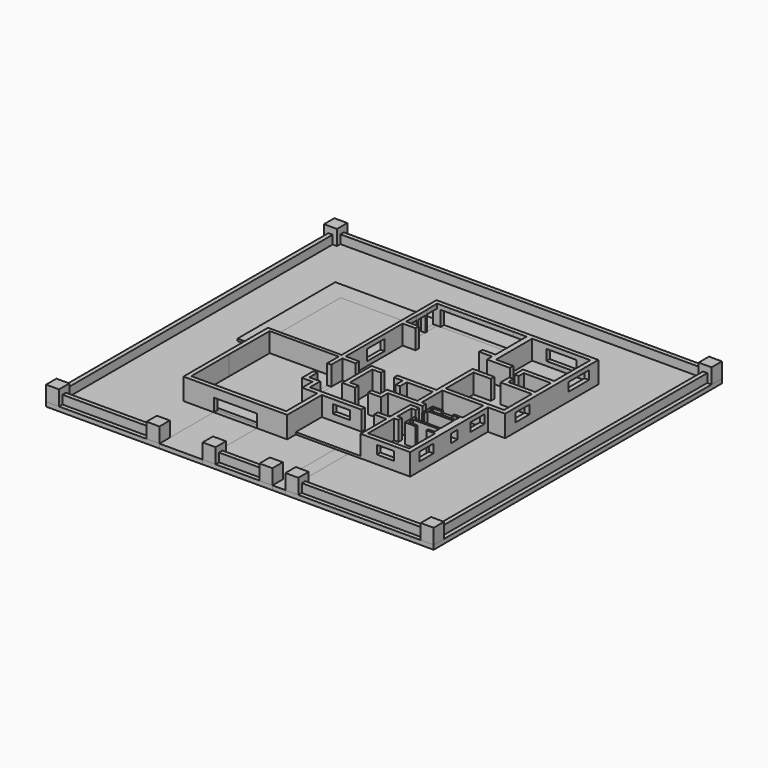
from build123d import *

# Parameters (mm, degrees)
F1_DEPTH  = 254
F2_DEPTH  = 254
F4_DEPTH  = 25.4
F5_W      = 203.2
F5_H      = 177.8
F6_DEPTH  = 50.8
F7_W      = 152.4
F7_H      = 254
F8_DEPTH  = 76.2
F9_W      = 939.5937236786
F9_H      = 25.4
F10_DEPTH = 53.34
F12_DEPTH = 63.5
F14_DEPTH = 76.2
F16_DEPTH = 101.6
F19_DEPTH = 76.2
F21_DEPTH = 76.2
F23_DEPTH = 76.2
F24_W     = 457.2
F24_H     = 177.8
F25_DEPTH = 76.2
F27_DEPTH = 76.2
F28_W     = 25.4
F28_H     = 50.8
F29_DEPTH = 50.8
F30_W     = 4055.1800727844
F30_H     = 3734.5069646835
F31_DEPTH = 50.8
F33_W     = 762
F33_H     = 1016
F34_DEPTH = 76.2
F35_W     = 762
F35_H     = 1016
F36_DEPTH = 76.2
F37_W     = 762
F37_H     = 1016
F38_DEPTH = 50.8
F39_DEPTH = 25.4
F40_DEPTH = 508
F41_DEPTH = 254
F42_DEPTH = 254
F45_DEPTH = 381
F46_W     = 152.4
F46_H     = 50.8
F47_DEPTH = 1016
F48_DEPTH = 1016
F49_W     = 152.4
F49_H     = 152.4
F50_DEPTH = 177.8
F52_DEPTH = 1524
F53_W     = 152.4
F53_H     = 152.4
F54_DEPTH = 177.8
F55_W     = 152.4
F55_H     = 152.4
F56_DEPTH = 177.8
F58_DEPTH = 3937
F60_DEPTH = 4318
F62_DEPTH = 4064
F65_DEPTH = 1905
F66_DEPTH = 1905
F67_DEPTH = 799.465
F68_W     = 508
F68_H     = 152.4
F69_DEPTH = 76.2
F70_W     = 152.4
F70_H     = 152.4
F71_DEPTH = 177.8
F72_DEPTH = 1143
F74_DEPTH = 635


with BuildPart() as f1:
    # F0 (on Top) → F1 (new body)
    with BuildSketch(Plane.XY):
        Polygon((177.8, 1192.7142027378), (-304.8, 1192.7142027378), (-635, 1192.7142027378), (-635, 508), (-635, -51.8857972622), (-47.8687277794, -51.8857972622), (587.1312722206, -51.8857972622), (587.1312722206, 456.1142027378), (1349.1312722206, 456.1142027378), (1349.1312722206, 75.1142027378), (1933.3312722206, 75.1142027378), (1933.3312722206, 1218.1142027378), (2136.5312722206, 1218.1142027378), (2136.5312722206, 2589.7142027378), (1349.1312722206, 2589.7142027378), (1179.474234581, 2589.7142027378), (431.8, 2589.7142027378), (231.5312722206, 2589.7142027378), (231.5312722206, 2081.7142027378), (231.5312722206, 1192.7142027378), align=None)
        Polygon((533.4, 0), (0, 0), (-584.2, 0), (-584.2, 558.8), (-581.2687277794, 1150.6002895355), (-301.8687277794, 1150.6002895355), (231.5312722206, 1150.6002895355), (231.5312722206, 608.5142027378), (355.6, 608.5142027378), (355.6, 456.1142027378), (482.6, 456.1142027378), (533.4, 456.1142027378), align=None, mode=Mode.SUBTRACT)
        Polygon((1396.7937236786, 127), (1396.7937236786, 508), (1447.5937236786, 508), (1447.5937236786, 558.8), (1396.7937236786, 558.8), (1396.7937236786, 762), (1447.5937236786, 762), (1447.5937236786, 812.8), (1396.7937236786, 812.8), (1345.9937236786, 812.8), (1345.9937236786, 762), (1345.9937236786, 508), (1041.1937236786, 508), (533.4, 508), (406.4, 508), (406.4, 660.4), (279.4, 660.4), (279.4, 1143), (437.7339612484, 1143), (437.7339612484, 1193.8), (279.4, 1193.8), (279.4, 2032), (431.8, 2032), (431.8, 2081.7142027378), (279.4, 2081.7142027378), (279.4, 2538.9142027378), (431.8, 2538.9142027378), (1179.474234581, 2540), (1331.874234581, 2540), (1331.874234581, 2081.7142027378), (1179.474234581, 2081.7142027378), (1179.474234581, 2032), (1331.874234581, 2032), (1331.874234581, 1957.4247688293), (1600.2, 1957.4247688293), (1600.2, 2008.2247688293), (1396.7937236786, 2008.2247688293), (1396.7937236786, 2540), (2082.5937236786, 2540), (2082.5937236786, 2008.2247688293), (1714.5, 2008.2247688293), (1714.5, 1957.4247688293), (1714.5, 1881.2247688293), (1765.3, 1881.2247688293), (1765.3, 1957.4247688293), (2082.5937236786, 1957.4247688293), (2082.5937236786, 1728.8247688293), (1765.3, 1728.8247688293), (1765.3, 1805.0247688293), (1714.5, 1805.0247688293), (1714.5, 1728.8247688293), (1714.5, 1678.0247688293), (2082.5937236786, 1678.0247688293), (2082.5937236786, 1270), (1828.5937236786, 1270), (1396.7937236786, 1270), (1396.7937236786, 1678.0247688293), (1600.2, 1678.0247688293), (1600.2, 1728.8247688293), (1345.9937236786, 1728.8247688293), (1345.9937236786, 1574.8), (1345.9937236786, 1320.8), (1345.9937236786, 1270), (1345.9937236786, 1193.8), (1193.5937236786, 1193.8), (1039.9870965004, 1193.8), (887.5870965004, 1193.8), (887.5870965004, 1143), (989.1870965004, 1143), (989.1870965004, 1041.4), (1039.9870965004, 1041.4), (1039.9870965004, 1143), (1193.5937236786, 1143), (1345.9937236786, 1143), (1345.9937236786, 1117.6073976807), (1345.9937236786, 939.8), (1345.9937236786, 914.4), (1039.9870965004, 914.4), (989.1870965004, 914.4), (989.1870965004, 812.8), (938.3870965004, 812.8), (887.5870965004, 812.8), (887.5870965004, 762), (1039.9870965004, 762), (1039.9870965004, 812.8), (1039.9870965004, 863.6), (1345.9937236786, 863.6), (1396.7937236786, 863.6), (1447.5937236786, 863.6), (1447.5937236786, 914.4), (1396.7937236786, 914.4), (1396.7937236786, 965.2), (1396.7937236786, 1219.2), (1828.5937236786, 1219.2), (1879.3937236786, 1219.2), (1879.3937236786, 914.4), (1879.3937236786, 811.3352970581), (1879.3937236786, 749.310195446), (1879.3937236786, 508), (1879.3937236786, 127), align=None, mode=Mode.SUBTRACT)
        Polygon((1777.7937236786, 508), (1879.3937236786, 508), (1879.3937236786, 749.310195446), (1879.3937236786, 811.3352970581), (1879.3937236786, 914.4), (1777.7937236786, 914.4), (1777.7937236786, 889), (1853.9937236786, 889), (1853.9937236786, 838.2), (1549.1937236786, 838.2), (1549.1937236786, 889), (1650.7937236786, 889), (1650.7937236786, 914.4), (1523.7937236786, 914.4), (1523.7937236786, 863.6), (1523.7937236786, 811.3352970581), (1523.7937236786, 757.4872970581), (1549.1937236786, 757.4872970581), (1549.1937236786, 811.3352970581), (1853.9937236786, 811.3352970581), (1853.9937236786, 622.3084970581), (1549.1937236786, 622.3084970581), (1549.1937236786, 650.748), (1523.7937236786, 650.748), (1523.7937236786, 596.9), (1523.7937236786, 508), (1650.7937236786, 508), (1650.7937236786, 533.4), (1549.1937236786, 533.4), (1549.1937236786, 596.9), (1853.9937236786, 596.9), (1853.9937236786, 533.4), (1777.7937236786, 533.4), align=None)
    extrude(amount=F1_DEPTH)

    # F0 (on Top) → F2 (join)
    with BuildSketch(Plane.XY):
        Polygon((177.8, 1192.7142027378), (-304.8, 1192.7142027378), (-635, 1192.7142027378), (-635, 508), (-635, -51.8857972622), (-47.8687277794, -51.8857972622), (587.1312722206, -51.8857972622), (587.1312722206, 456.1142027378), (1349.1312722206, 456.1142027378), (1349.1312722206, 75.1142027378), (1933.3312722206, 75.1142027378), (1933.3312722206, 1218.1142027378), (2136.5312722206, 1218.1142027378), (2136.5312722206, 2589.7142027378), (1349.1312722206, 2589.7142027378), (1179.474234581, 2589.7142027378), (431.8, 2589.7142027378), (231.5312722206, 2589.7142027378), (231.5312722206, 2081.7142027378), (231.5312722206, 1192.7142027378), align=None)
        Polygon((533.4, 0), (0, 0), (-584.2, 0), (-584.2, 558.8), (-581.2687277794, 1150.6002895355), (-301.8687277794, 1150.6002895355), (231.5312722206, 1150.6002895355), (231.5312722206, 608.5142027378), (355.6, 608.5142027378), (355.6, 456.1142027378), (482.6, 456.1142027378), (533.4, 456.1142027378), align=None, mode=Mode.SUBTRACT)
        Polygon((1396.7937236786, 127), (1396.7937236786, 508), (1447.5937236786, 508), (1447.5937236786, 558.8), (1396.7937236786, 558.8), (1396.7937236786, 762), (1447.5937236786, 762), (1447.5937236786, 812.8), (1396.7937236786, 812.8), (1345.9937236786, 812.8), (1345.9937236786, 762), (1345.9937236786, 508), (1041.1937236786, 508), (533.4, 508), (406.4, 508), (406.4, 660.4), (279.4, 660.4), (279.4, 1143), (437.7339612484, 1143), (437.7339612484, 1193.8), (279.4, 1193.8), (279.4, 2032), (431.8, 2032), (431.8, 2081.7142027378), (279.4, 2081.7142027378), (279.4, 2538.9142027378), (431.8, 2538.9142027378), (1179.474234581, 2540), (1331.874234581, 2540), (1331.874234581, 2081.7142027378), (1179.474234581, 2081.7142027378), (1179.474234581, 2032), (1331.874234581, 2032), (1331.874234581, 1957.4247688293), (1600.2, 1957.4247688293), (1600.2, 2008.2247688293), (1396.7937236786, 2008.2247688293), (1396.7937236786, 2540), (2082.5937236786, 2540), (2082.5937236786, 2008.2247688293), (1714.5, 2008.2247688293), (1714.5, 1957.4247688293), (1714.5, 1881.2247688293), (1765.3, 1881.2247688293), (1765.3, 1957.4247688293), (2082.5937236786, 1957.4247688293), (2082.5937236786, 1728.8247688293), (1765.3, 1728.8247688293), (1765.3, 1805.0247688293), (1714.5, 1805.0247688293), (1714.5, 1728.8247688293), (1714.5, 1678.0247688293), (2082.5937236786, 1678.0247688293), (2082.5937236786, 1270), (1828.5937236786, 1270), (1396.7937236786, 1270), (1396.7937236786, 1678.0247688293), (1600.2, 1678.0247688293), (1600.2, 1728.8247688293), (1345.9937236786, 1728.8247688293), (1345.9937236786, 1574.8), (1345.9937236786, 1320.8), (1345.9937236786, 1270), (1345.9937236786, 1193.8), (1193.5937236786, 1193.8), (1039.9870965004, 1193.8), (887.5870965004, 1193.8), (887.5870965004, 1143), (989.1870965004, 1143), (989.1870965004, 1041.4), (1039.9870965004, 1041.4), (1039.9870965004, 1143), (1193.5937236786, 1143), (1345.9937236786, 1143), (1345.9937236786, 1117.6073976807), (1345.9937236786, 939.8), (1345.9937236786, 914.4), (1039.9870965004, 914.4), (989.1870965004, 914.4), (989.1870965004, 812.8), (938.3870965004, 812.8), (887.5870965004, 812.8), (887.5870965004, 762), (1039.9870965004, 762), (1039.9870965004, 812.8), (1039.9870965004, 863.6), (1345.9937236786, 863.6), (1396.7937236786, 863.6), (1447.5937236786, 863.6), (1447.5937236786, 914.4), (1396.7937236786, 914.4), (1396.7937236786, 965.2), (1396.7937236786, 1219.2), (1828.5937236786, 1219.2), (1879.3937236786, 1219.2), (1879.3937236786, 914.4), (1879.3937236786, 811.3352970581), (1879.3937236786, 749.310195446), (1879.3937236786, 508), (1879.3937236786, 127), align=None, mode=Mode.SUBTRACT)
    extrude(amount=F2_DEPTH)

    # F5 (on face) → F6 (cut)
    with BuildSketch(Plane(origin=(231.5312722206, 0, 0), x_dir=(0, -1, 0), z_dir=(-1, 0, 0))):
        Polygon((-777.9572461367, 203.2), (-777.9572461367, 254), (-879.5572461367, 254), (-981.1572461367, 254), (-981.1572461367, 203.2), align=None)
        with Locations((-879.5572461367, 114.3)):
            Rectangle(F5_W, F5_H)
    extrude(amount=-F6_DEPTH, mode=Mode.SUBTRACT)

    # F7 (on face) → F8 (cut)
    with BuildSketch(Plane.XZ.offset(-456.1142027378)):
        with Locations((1128.791085434, 127)):
            Rectangle(F7_W, F7_H)
    extrude(amount=-F8_DEPTH, mode=Mode.SUBTRACT)

    # F11 (on face) → F12 (cut)
    with BuildSketch(Plane.XZ.offset(-456.1142027378)):
        Polygon((921.4611788273, 203.2), (819.8611788273, 203.2), (718.2611788273, 203.2), (718.2611788273, 101.6), (921.4611788273, 101.6), align=None)
    extrude(amount=-F12_DEPTH, mode=Mode.SUBTRACT)

    # F13 (on face) → F14 (cut)
    with BuildSketch(Plane.XZ.offset(-75.1142027378)):
        Polygon((1742.8312722206, 203.2), (1641.2312722206, 203.2), (1539.6312722206, 203.2), (1539.6312722206, 101.6), (1742.8312722206, 101.6), align=None)
    extrude(amount=-F14_DEPTH, mode=Mode.SUBTRACT)

    # F15 (on face) → F16 (cut)
    with BuildSketch(Plane.YZ.offset(1933.3312722206)):
        Polygon((418.0142027378, 203.2), (316.4142027378, 203.2), (214.8142027378, 203.2), (214.8142027378, 101.6), (418.0142027378, 101.6), align=None)
        Polygon((1167.3142027378, 203.2), (1065.7142027378, 203.2), (964.1142027378, 203.2), (964.1142027378, 101.6), (1167.3142027378, 101.6), align=None)
        Polygon((773.6142027378, 203.2), (710.1142027378, 203.2), (672.0142027378, 203.2), (672.0142027378, 101.6), (773.6142027378, 101.6), align=None)
    extrude(amount=-F16_DEPTH, mode=Mode.SUBTRACT)

    # F18 (on face) → F19 (cut)
    with BuildSketch(Plane.YZ.offset(2136.5312722206)):
        Polygon((2452.1544022799, 203.2), (2299.7544022799, 203.2), (2147.3544022799, 203.2), (2147.3544022799, 101.6), (2452.1544022799, 101.6), align=None)
        Polygon((1573.7142027378, 203.2), (1472.1142027378, 203.2), (1370.5142027378, 203.2), (1370.5142027378, 101.6), (1573.7142027378, 101.6), align=None)
    extrude(amount=-F19_DEPTH, mode=Mode.SUBTRACT)

    # F20 (on face) → F21 (cut)
    with BuildSketch(Plane(origin=(0, 2589.7142027378, 0), x_dir=(-1, 0, 0), z_dir=(0, 1, 0))):
        Polygon((-1565.0312722206, 203.2), (-1742.8312722206, 203.2), (-1920.6312722206, 203.2), (-1920.6312722206, 76.2), (-1565.0312722206, 76.2), align=None)
    extrude(amount=-F21_DEPTH, mode=Mode.SUBTRACT)

    # F22 (on face) → F23 (cut)
    with BuildSketch(Plane(origin=(0, 2589.7142027378, 0), x_dir=(-1, 0, 0), z_dir=(0, 1, 0))):
        Polygon((-320.4312722206, 203.2), (-803.0312722206, 203.2), (-1285.6312722206, 203.2), (-1285.6312722206, 25.4), (-320.4312722206, 25.4), align=None)
    extrude(amount=-F23_DEPTH, mode=Mode.SUBTRACT)

    # F24 (on face) → F25 (cut)
    with BuildSketch(Plane(origin=(231.5312722206, 0, 0), x_dir=(0, -1, 0), z_dir=(-1, 0, 0))):
        with Locations((-2310.3142027378, 114.3)):
            Rectangle(F24_W, F24_H)
    extrude(amount=-F25_DEPTH, mode=Mode.SUBTRACT)

    # F26 (on face) → F27 (cut)
    with BuildSketch(Plane(origin=(231.5312722206, 0, 0), x_dir=(0, -1, 0), z_dir=(-1, 0, 0))):
        Polygon((-1510.2142027378, 203.2), (-1764.2142027378, 203.2), (-1764.2142027378, 76.2), (-1637.2142027378, 76.2), (-1510.2142027378, 76.2), align=None)
    extrude(amount=-F27_DEPTH, mode=Mode.SUBTRACT)



with BuildPart() as f2:
    # F0 (on Top) → F2, piece 2 (new body)
    with BuildSketch(Plane.XY):
        Polygon((582.7870965004, 762), (735.1870965004, 762), (735.1870965004, 812.8), (633.5870965004, 812.8), (633.5870965004, 1143), (735.1870965004, 1143), (735.1870965004, 1193.8), (582.7870965004, 1193.8), (582.7870965004, 1143), (582.7870965004, 812.8), align=None)
    extrude(amount=F2_DEPTH)


with BuildPart() as f4:
    # F3 (on face) → F4 (new body)
    with BuildSketch(Plane(origin=(0, 0, 0), x_dir=(1, 0, 0), z_dir=(0, 0, -1))):
        Polygon((533.4, -456.1142027378), (533.4, 0), (-584.2, 0), (-584.2, -558.8), (-581.2687277794, -1150.6002895355), (231.5312722206, -1150.6002895355), (231.5312722206, -608.5142027378), (355.6, -608.5142027378), (355.6, -456.1142027378), align=None)
    extrude(amount=-F4_DEPTH)


with BuildPart() as f4b:
    # F3 (on face) → F4, piece 2 (new body)
    with BuildSketch(Plane(origin=(0, 0, 0), x_dir=(1, 0, 0), z_dir=(0, 0, -1))):
        Polygon((1039.9870965004, -762), (1039.9870965004, -863.6), (1447.5937236786, -863.6), (1447.5937236786, -914.4), (1396.7937236786, -914.4), (1396.7937236786, -1219.2), (1879.3937236786, -1219.2), (1879.3937236786, -914.4), (1777.7937236786, -914.4), (1777.7937236786, -889), (1853.9937236786, -889), (1853.9937236786, -838.2), (1549.1937236786, -838.2), (1549.1937236786, -889), (1650.7937236786, -889), (1650.7937236786, -914.4), (1523.7937236786, -914.4), (1523.7937236786, -757.4872970581), (1549.1937236786, -757.4872970581), (1549.1937236786, -811.3352970581), (1853.9937236786, -811.3352970581), (1853.9937236786, -622.3084970581), (1549.1937236786, -622.3084970581), (1549.1937236786, -650.748), (1523.7937236786, -650.748), (1523.7937236786, -508), (1650.7937236786, -508), (1650.7937236786, -533.4), (1549.1937236786, -533.4), (1549.1937236786, -596.9), (1853.9937236786, -596.9), (1853.9937236786, -533.4), (1777.7937236786, -533.4), (1777.7937236786, -508), (1879.3937236786, -508), (1879.3937236786, -127), (1396.7937236786, -127), (1396.7937236786, -508), (1447.5937236786, -508), (1447.5937236786, -558.8), (1396.7937236786, -558.8), (1396.7937236786, -762), (1447.5937236786, -762), (1447.5937236786, -812.8), (1345.9937236786, -812.8), (1345.9937236786, -508), (406.4, -508), (406.4, -660.4), (279.4, -660.4), (279.4, -1143), (437.7339612484, -1143), (437.7339612484, -1193.8), (279.4, -1193.8), (279.4, -2032), (431.8, -2032), (431.8, -2081.7142027378), (279.4, -2081.7142027378), (279.4, -2538.9142027378), (431.8, -2538.9142027378), (1179.474234581, -2540), (1331.874234581, -2540), (1331.874234581, -2081.7142027378), (1179.474234581, -2081.7142027378), (1179.474234581, -2032), (1331.874234581, -2032), (1331.874234581, -1957.4247688293), (1600.2, -1957.4247688293), (1600.2, -2008.2247688293), (1396.7937236786, -2008.2247688293), (1396.7937236786, -2540), (2082.5937236786, -2540), (2082.5937236786, -2008.2247688293), (1714.5, -2008.2247688293), (1714.5, -1881.2247688293), (1765.3, -1881.2247688293), (1765.3, -1957.4247688293), (2082.5937236786, -1957.4247688293), (2082.5937236786, -1728.8247688293), (1765.3, -1728.8247688293), (1765.3, -1805.0247688293), (1714.5, -1805.0247688293), (1714.5, -1678.0247688293), (2082.5937236786, -1678.0247688293), (2082.5937236786, -1270), (1396.7937236786, -1270), (1396.7937236786, -1678.0247688293), (1600.2, -1678.0247688293), (1600.2, -1728.8247688293), (1345.9937236786, -1728.8247688293), (1345.9937236786, -1193.8), (887.5870965004, -1193.8), (887.5870965004, -1143), (989.1870965004, -1143), (989.1870965004, -1041.4), (1039.9870965004, -1041.4), (1039.9870965004, -1143), (1345.9937236786, -1143), (1345.9937236786, -914.4), (989.1870965004, -914.4), (989.1870965004, -812.8), (887.5870965004, -812.8), (887.5870965004, -762), align=None)
    extrude(amount=-F4_DEPTH)


with BuildPart() as f10:
    # F9 (on face) → F10 (new body)
    with BuildSketch(Plane.XZ.offset(-508)):
        with Locations((876.1968618393, 12.7)):
            Rectangle(F9_W, F9_H)
    extrude(amount=F10_DEPTH)


with BuildPart() as f29:
    # F28 (on face) → F29 (new body)
    with BuildSketch(Plane(origin=(231.5312722206, 0, 0), x_dir=(0, -1, 0), z_dir=(-1, 0, 0))):
        Polygon((-2361.1142027378, 254), (-2361.1142027378, 203.2), (-2310.3142027378, 203.2), (-2259.5142027378, 203.2), (-2259.5142027378, 254), align=None)
        Polygon((-2361.1142027378, 25.4), (-2361.1142027378, 203.2), (-2386.5142027378, 203.2), (-2386.5142027378, 0), (-2259.5142027378, 0), (-2259.5142027378, 25.4), (-2310.3142027378, 25.4), align=None)
        with Locations((-2373.8142027378, 228.6)):
            Rectangle(F28_W, F28_H)
        with Locations((-2246.8142027378, 228.6)):
            Rectangle(F28_W, F28_H)
        Polygon((-2234.1142027378, 203.2), (-2259.5142027378, 203.2), (-2259.5142027378, 25.4), (-2259.5142027378, 0), (-2234.1142027378, 0), align=None)
    extrude(amount=-F29_DEPTH)


with BuildPart() as f31:
    # F30 (on face) → F31 (new body)
    with BuildSketch(Plane(origin=(0, 0, 0), x_dir=(1, 0, 0), z_dir=(0, 0, -1))):
        with Locations((922.8382110596, -1270.1082825661)):
            Rectangle(F30_W, F30_H)
        Polygon((2136.5312722206, -2589.7142027378), (231.5312722206, -2589.7142027378), (231.5312722206, -1192.7142027378), (-635, -1192.7142027378), (-635, 51.8857972622), (587.1312722206, 51.8857972622), (587.1312722206, -456.1142027378), (1052.591085434, -456.1142027378), (1052.591085434, -508), (406.4, -508), (406.4, -660.4), (279.4, -660.4), (279.4, -1143), (437.7339612484, -1143), (437.7339612484, -1193.8), (279.4, -1193.8), (279.4, -2032), (431.8, -2032), (431.8, -2081.7142027378), (279.4, -2081.7142027378), (279.4, -2538.9142027378), (431.8, -2538.9142027378), (1179.474234581, -2540), (1331.874234581, -2540), (1331.874234581, -2081.7142027378), (1179.474234581, -2081.7142027378), (1179.474234581, -2032), (1331.874234581, -2032), (1331.874234581, -1957.4247688293), (1600.2, -1957.4247688293), (1600.2, -2008.2247688293), (1396.7937236786, -2008.2247688293), (1396.7937236786, -2540), (2082.5937236786, -2540), (2082.5937236786, -2008.2247688293), (1714.5, -2008.2247688293), (1714.5, -1881.2247688293), (1765.3, -1881.2247688293), (1765.3, -1957.4247688293), (2082.5937236786, -1957.4247688293), (2082.5937236786, -1728.8247688293), (1765.3, -1728.8247688293), (1765.3, -1805.0247688293), (1714.5, -1805.0247688293), (1714.5, -1678.0247688293), (2082.5937236786, -1678.0247688293), (2082.5937236786, -1270), (1396.7937236786, -1270), (1396.7937236786, -1678.0247688293), (1600.2, -1678.0247688293), (1600.2, -1728.8247688293), (1345.9937236786, -1728.8247688293), (1345.9937236786, -1193.8), (887.5870965004, -1193.8), (887.5870965004, -1143), (989.1870965004, -1143), (989.1870965004, -1041.4), (1039.9870965004, -1041.4), (1039.9870965004, -1143), (1345.9937236786, -1143), (1345.9937236786, -914.4), (989.1870965004, -914.4), (989.1870965004, -812.8), (887.5870965004, -812.8), (887.5870965004, -762), (1039.9870965004, -762), (1039.9870965004, -863.6), (1447.5937236786, -863.6), (1447.5937236786, -914.4), (1396.7937236786, -914.4), (1396.7937236786, -1219.2), (1879.3937236786, -1219.2), (1879.3937236786, -914.4), (1777.7937236786, -914.4), (1777.7937236786, -889), (1853.9937236786, -889), (1853.9937236786, -838.2), (1549.1937236786, -838.2), (1549.1937236786, -889), (1650.7937236786, -889), (1650.7937236786, -914.4), (1523.7937236786, -914.4), (1523.7937236786, -757.4872970581), (1549.1937236786, -757.4872970581), (1549.1937236786, -811.3352970581), (1853.9937236786, -811.3352970581), (1853.9937236786, -622.3084970581), (1549.1937236786, -622.3084970581), (1549.1937236786, -650.748), (1523.7937236786, -650.748), (1523.7937236786, -508), (1650.7937236786, -508), (1650.7937236786, -533.4), (1549.1937236786, -533.4), (1549.1937236786, -596.9), (1853.9937236786, -596.9), (1853.9937236786, -533.4), (1777.7937236786, -533.4), (1777.7937236786, -508), (1879.3937236786, -508), (1879.3937236786, -127), (1396.7937236786, -127), (1396.7937236786, -508), (1447.5937236786, -508), (1447.5937236786, -558.8), (1396.7937236786, -558.8), (1396.7937236786, -762), (1447.5937236786, -762), (1447.5937236786, -812.8), (1345.9937236786, -812.8), (1345.9937236786, -508), (1204.991085434, -508), (1204.991085434, -456.1142027378), (1349.1312722206, -456.1142027378), (1349.1312722206, -75.1142027378), (1933.3312722206, -75.1142027378), (1933.3312722206, -1218.1142027378), (2136.5312722206, -1218.1142027378), align=None, mode=Mode.SUBTRACT)
    extrude(amount=F31_DEPTH)

    # F33 (on face) → F34 (cut)
    with BuildSketch(Plane.XY):
        with Locations((-381, 1911.4676551819)):
            Rectangle(F33_W, F33_H)
    extrude(amount=-F34_DEPTH, mode=Mode.SUBTRACT)

    # F40 (add): a face of the model
    f40_faces = [f31.faces().sort_by_distance(p)[0] for p in [
        (-1104.7518253326, 1270.1082825661, -25.4),
    ]]
    extrude(f40_faces, amount=F40_DEPTH)

    # F41 (add): a face of the model
    f41_faces = [f31.faces().sort_by_distance(p)[0] for p in [
        (668.8382110596, -597.1451997757, -25.4),
    ]]
    extrude(f41_faces, amount=F41_DEPTH)

    # F42 (add): a face of the model
    f42_faces = [f31.faces().sort_by_distance(p)[0] for p in [
        (668.8382110596, 3137.3617649078, -25.4),
    ]]
    extrude(f42_faces, amount=F42_DEPTH)

    # F46 (on face) → F47 (cut)
    with BuildSketch(Plane.XZ.offset(851.1451997757)):
        with Locations((1128.791085434, -25.4)):
            Rectangle(F46_W, F46_H)
    extrude(amount=-F47_DEPTH, mode=Mode.SUBTRACT)


with BuildPart() as f31b:
    # F30 (on face) → F31, piece 2 (new body)
    with BuildSketch(Plane(origin=(0, 0, 0), x_dir=(1, 0, 0), z_dir=(0, 0, -1))):
        Polygon((533.4, -456.1142027378), (533.4, 0), (-584.2, 0), (-584.2, -558.8), (-581.2687277794, -1150.6002895355), (231.5312722206, -1150.6002895355), (231.5312722206, -608.5142027378), (355.6, -608.5142027378), (355.6, -456.1142027378), align=None)
    extrude(amount=F31_DEPTH)


with BuildPart() as f36:
    # F35 (on face) → F36 (new body)
    with BuildSketch(Plane(origin=(0, 0, -50.8), x_dir=(1, 0, 0), z_dir=(0, 0, -1))):
        with Locations((-381, -1911.4676551819)):
            Rectangle(F35_W, F35_H)
    extrude(amount=-F36_DEPTH)


with BuildPart() as f38:
    # F37 (on face) → F38 (new body)
    with BuildSketch(Plane.XY):
        Polygon((231.5312722206, 1192.7142027378), (231.5312722206, 2589.7142027378), (231.5312722206, 2630.2114551819), (-993.521, 2630.2114551819), (-993.521, 2419.4676551819), (-993.521, 1192.7142027378), (-762, 1192.7142027378), (-635, 1192.7142027378), align=None)
        with Locations((-381, 1911.4676551819)):
            Rectangle(F37_W, F37_H, mode=Mode.SUBTRACT)
    extrude(amount=-F38_DEPTH)


with BuildPart() as f39:
    # F39 (new): a face of the model
    f39_faces = [f38.part.faces().sort_by_distance(p)[0] for p in [
        (212.6443682381, 1911.4628289598, 0),
    ]]
    extrude(f39_faces, amount=F39_DEPTH)


with BuildPart() as f45:
    # F44 (on face) → F45 (new body)
    with BuildSketch(Plane.XZ.offset(-454.66)):
        Polygon((1345.9937236786, 25.4), (587.1312722206, 25.4), (587.1312722206, 0), (1345.9937236786, 0), (1349.1312722206, 0), (1349.1312722206, 25.4), align=None)
    extrude(amount=F45_DEPTH)


with BuildPart() as f48:
    # F48 (new): a face of the model
    f48_faces = [f31.part.faces().sort_by_distance(p)[0] for p in [
        (1128.791085434, 164.8548002243, -25.4),
    ]]
    extrude(f48_faces, amount=F48_DEPTH)


with BuildPart() as f50:
    # F49 (on face) → F50 (new body)
    with BuildSketch(Plane.XY):
        with Locations((976.391085434, -774.9451997757)):
            Rectangle(F49_W, F49_H)
    extrude(amount=F50_DEPTH)


with BuildPart() as f50b:
    # F49 (on face) → F50, piece 2 (new body)
    with BuildSketch(Plane.XY):
        with Locations((1281.191085434, -774.9451997757)):
            Rectangle(F49_W, F49_H)
    extrude(amount=F50_DEPTH)


with BuildPart() as f52:
    # F51 (on face) → F52 (new body)
    with BuildSketch(Plane.YZ.offset(1357.391085434)):
        Polygon((-800.3451997757, 101.6), (-800.3451997757, 0), (-774.9451997757, 0), (-749.5451997757, 0), (-749.5451997757, 101.6), align=None)
    extrude(amount=F52_DEPTH)


with BuildPart() as f54:
    # F53 (on face) → F54 (new body)
    with BuildSketch(Plane.XY):
        with Locations((2874.2282474518, -774.9451997757)):
            Rectangle(F53_W, F53_H)
    extrude(amount=F54_DEPTH)


with BuildPart() as f56:
    # F55 (on face) → F56 (new body)
    with BuildSketch(Plane.XY):
        with Locations((2874.2282474518, 3315.1617649078)):
            Rectangle(F55_W, F55_H)
    extrude(amount=F56_DEPTH)


with BuildPart() as f56b:
    # F55 (on face) → F56, piece 2 (new body)
    with BuildSketch(Plane.XY):
        with Locations((-1536.5518253326, 3315.1617649078)):
            Rectangle(F55_W, F55_H)
    extrude(amount=F56_DEPTH)


with BuildPart() as f56c:
    # F55 (on face) → F56, piece 3 (new body)
    with BuildSketch(Plane.XY):
        with Locations((-1536.5518253326, -774.9451997757)):
            Rectangle(F55_W, F55_H)
    extrude(amount=F56_DEPTH)


with BuildPart() as f58:
    # F57 (on face) → F58 (new body)
    with BuildSketch(Plane.XZ.offset(-3238.9617649078)):
        Polygon((2848.8282474518, 101.6), (2848.8282474518, 0), (2874.2282474518, 0), (2899.6282474518, 0), (2899.6282474518, 101.6), align=None)
    extrude(amount=F58_DEPTH)


with BuildPart() as f60:
    # F59 (on face) → F60 (new body)
    with BuildSketch(Plane.YZ.offset(-1460.3518253326)):
        Polygon((3289.7617649078, 0), (3315.1617649078, 0), (3340.5617649078, 0), (3340.5617649078, 101.6), (3289.7617649078, 101.6), align=None)
    extrude(amount=F60_DEPTH)


with BuildPart() as f62:
    # F61 (on face) → F62 (new body)
    with BuildSketch(Plane.XZ.offset(-3238.9617649078)):
        Polygon((-1561.9518253326, 0), (-1536.5518253326, 0), (-1511.1518253326, 0), (-1511.1518253326, 101.6), (-1561.9518253326, 101.6), align=None)
    extrude(amount=F62_DEPTH)


with BuildPart() as f1_1:
    add(f1.part)

    add(f31.part)  # F65 merges F31
    # F64 (on face) → F65 (join)
    with BuildSketch(Plane.XZ.offset(51.8857972622)):
        Polygon((230.0656361103, 0), (-23.9343638897, 0), (-277.9343638897, 0), (-277.9343638897, -50.8), (230.0656361103, -50.8), align=None)
    extrude(amount=F65_DEPTH)

    # F66 (cut): a face of the model
    f66_faces = [f1_1.faces().sort_by_distance(p)[0] for p in [
        (-23.9343638897, -1956.8857972622, -25.4),
    ]]
    extrude(f66_faces, amount=-F66_DEPTH, mode=Mode.SUBTRACT)

    # F68 (on face) → F69 (cut)
    with BuildSketch(Plane.XZ.offset(51.8857972622)):
        with Locations((-23.9343638897, 76.2)):
            Rectangle(F68_W, F68_H)
    extrude(amount=-F69_DEPTH, mode=Mode.SUBTRACT)


with BuildPart() as f67:
    # F64 (on face) → F67 (new body)
    with BuildSketch(Plane.XZ.offset(51.8857972622)):
        Polygon((230.0656361103, 0), (-23.9343638897, 0), (-277.9343638897, 0), (-277.9343638897, -50.8), (230.0656361103, -50.8), align=None)
    extrude(amount=F67_DEPTH)


with BuildPart() as f71:
    # F70 (on face) → F71 (new body)
    with BuildSketch(Plane.XY):
        with Locations((-354.1343638897, -774.9451997757)):
            Rectangle(F70_W, F70_H)
    extrude(amount=F71_DEPTH)


with BuildPart() as f71b:
    # F70 (on face) → F71, piece 2 (new body)
    with BuildSketch(Plane.XY):
        with Locations((306.2656361103, -774.9451997757)):
            Rectangle(F70_W, F70_H)
    extrude(amount=F71_DEPTH)


with BuildPart() as f72:
    # F63 (on face) → F72 (new body)
    with BuildSketch(Plane.YZ.offset(-1460.3518253326)):
        Polygon((-800.3451997757, 0), (-774.9451997757, 0), (-749.5451997757, 0), (-749.5451997757, 101.6), (-800.3451997757, 101.6), align=None)
    extrude(amount=F72_DEPTH)


with BuildPart() as f74:
    # F73 (on face) → F74 (new body)
    with BuildSketch(Plane.YZ.offset(382.4656361103)):
        Polygon((-800.3451997757, 0), (-774.9451997757, 0), (-749.5451997757, 0), (-749.5451997757, 101.6), (-800.3451997757, 101.6), align=None)
    extrude(amount=F74_DEPTH)


solid = Compound([f2.part, f4.part, f4b.part, f10.part, f29.part, f31b.part, f36.part, f38.part, f39.part, f45.part, f48.part, f50.part, f50b.part, f52.part, f54.part, f56.part, f56b.part, f56c.part, f58.part, f60.part, f62.part, f1_1.part, f67.part, f71.part, f71b.part, f72.part, f74.part])
